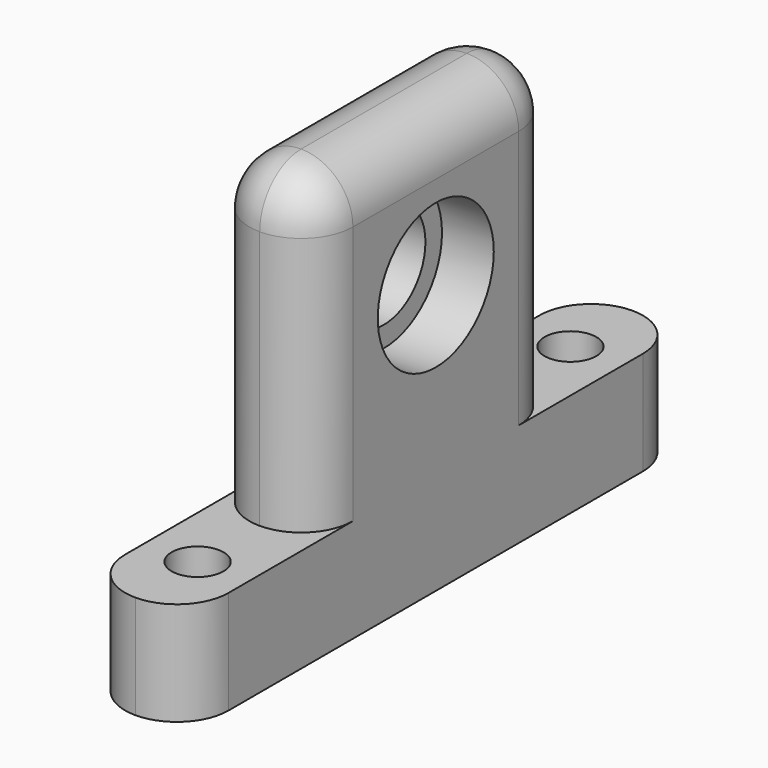
from build123d import *

# Parameters (mm, degrees)
F0_W     = 10
F0_H     = 30
F1_DEPTH = 40
F0_H_2   = 15
F0_R     = 2.5
F2_DEPTH = 10
F3_R     = 5
F4_DEPTH = 25
F3_R_2   = 7
F5_DEPTH = 5
F6_R     = 4.99999
F7_R     = 4.99999


# Not quite as in the source:
# - a fillet or chamfer is up to 0.001 mm smaller than in the source, because OpenCascade refuses the exact size


with BuildPart() as f1:
    # F0 (on Top) → F1 (new body)
    with BuildSketch(Plane.XY):
        with Locations((0, -15)):
            Rectangle(F0_W, F0_H)
    extrude(amount=F1_DEPTH)

    # F0 (on Top) → F2 (join)
    with BuildSketch(Plane.XY):
        with Locations((0, 7.5)):
            Rectangle(F0_W, F0_H_2)
        with Locations((0, 7.5)):
            Circle(F0_R, mode=Mode.SUBTRACT)
        with Locations((0, -37.5)):
            Rectangle(F0_W, F0_H_2)
        with Locations((0, -37.5)):
            Circle(F0_R, mode=Mode.SUBTRACT)
    extrude(amount=F2_DEPTH)

    # F3 (on face) → F4 (cut)
    with BuildSketch(Plane.YZ.offset(5)):
        with Locations((-15, 26)):
            Circle(F3_R)
    extrude(amount=-F4_DEPTH, mode=Mode.SUBTRACT)

    # F3 (on face) → F5 (cut)
    with BuildSketch(Plane.YZ.offset(5)):
        with Locations((-15, 26)):
            Circle(F3_R_2)
        with Locations((-15, 26)):
            Circle(F3_R, mode=Mode.SUBTRACT)
    extrude(amount=-F5_DEPTH, mode=Mode.SUBTRACT)

    # F6 (radius 5 in the source; OpenCascade refuses exactly that, so slightly less here)
    f6_edges = [f1.edges().sort_by_distance(p)[0] for p in [
        (0, -30, 40),
        (5, -15, 40),
        (0, 0, 40),
        (-5, -15, 40),
        (5, 0, 25),
        (5, -30, 25),
        (-5, -30, 25),
        (-5, 0, 25),
    ]]
    fillet(f6_edges, radius=F6_R)

    # F7 (radius 5 in the source; OpenCascade refuses exactly that, so slightly less here)
    f7_edges = [f1.edges().sort_by_distance(p)[0] for p in [
        (5, 15, 5),
        (-5, 15, 5),
        (5, -45, 5),
        (-5, -45, 5),
    ]]
    fillet(f7_edges, radius=F7_R)


solid = f1.part
